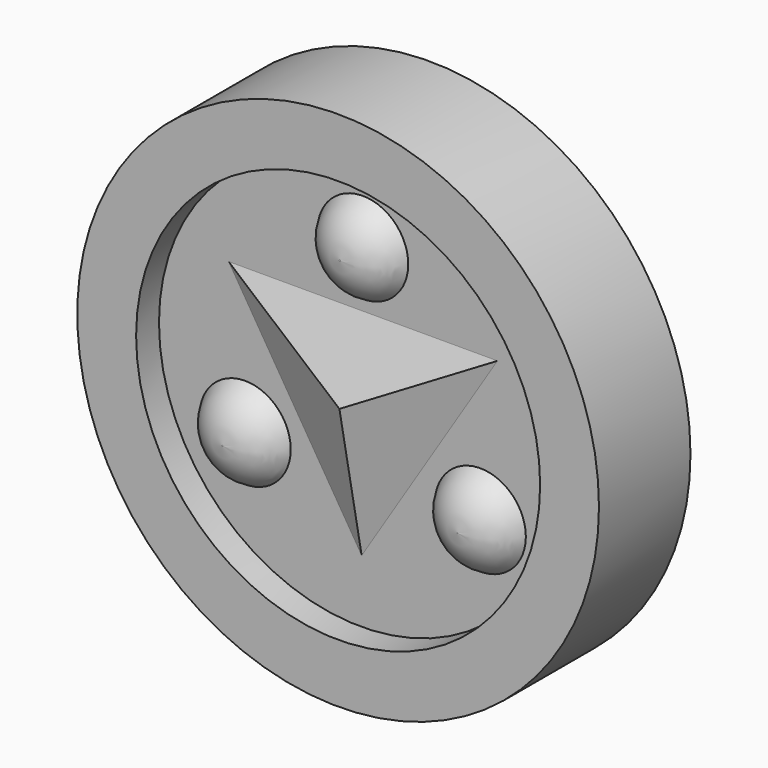
from build123d import *

# Parameters (mm, degrees)
F0_R          = 57.9269385224
F0_R_2        = 45.238930614
F0_R_3        = 10.232456426
F0_R_4        = 9.9260337363
F0_R_5        = 10.3400506536
F1_DEPTH      = 12.7
F2_DEPTH      = 12.7
F3_R          = 44.8601198224
F4_DEPTH      = 6.35
F5_R          = 44.7159015694
F6_DEPTH      = 6.35
F8_DEPTH      = 6.35
F10_DEPTH     = 6.35
F11_R         = 10.0879812564
F11_R_2       = 10.1077702508
F11_R_3       = 10.130036121
F12_DEPTH     = 6.35
F16_T4_DEPTH  = 143.3938123808
F16_T11_DEPTH = 146.5521785494
F16_T18_DEPTH = 143.0711301992


# Not quite as in the source:
# - a fillet or chamfer that OpenCascade refuses, or shapes differently, is made with other operations: its cross-section is extruded or revolved along the edge and cut away or added


with BuildPart() as f1:
    # F0 (on Front) → F1 (new body)
    with BuildSketch(Plane.XZ):
        Circle(F0_R)
        Circle(F0_R_2, mode=Mode.SUBTRACT)
        Circle(F0_R_2)
        with Locations((-26.1295642704, -15.3669575229)):
            Circle(F0_R_3, mode=Mode.SUBTRACT)
        Polygon((-12.544834055, -34.5090515912), (0, -5.3877583705), (12.6424450427, -34.5090515912), align=None, mode=Mode.SUBTRACT)
        with Locations((26.1333119124, -15.1850637048)):
            Circle(F0_R_4, mode=Mode.SUBTRACT)
        Polygon((-36.0336452723, 4.8764180392), (-24.01153557, 26.9035063684), (-4.5260344632, 1.7700339667), align=None, mode=Mode.SUBTRACT)
        Polygon((36.1581519246, 4.842239432), (4.4649434276, 1.758374623), (24.0084677935, 26.875147596), align=None, mode=Mode.SUBTRACT)
        with Locations((0, 29.5979101211)):
            Circle(F0_R_5, mode=Mode.SUBTRACT)
        with Locations((0, 29.5979101211)):
            Circle(F0_R_5)
        Polygon((-4.5260344632, 1.7700339667), (-24.01153557, 26.9035063684), (-36.0336452723, 4.8764180392), align=None)
        with Locations((-26.1295642704, -15.3669575229)):
            Circle(F0_R_3)
        Polygon((12.6424450427, -34.5090515912), (0, -5.3877583705), (-12.544834055, -34.5090515912), align=None)
        with Locations((26.1333119124, -15.1850637048)):
            Circle(F0_R_4)
        Polygon((24.0084677935, 26.875147596), (4.4649434276, 1.758374623), (36.1581519246, 4.842239432), align=None)
    extrude(amount=F1_DEPTH)

    # F2 (add): a face of the model
    f2_faces = [f1.faces().sort_by_distance(p)[0] for p in [
        (0, 0, 0),
    ]]
    extrude(f2_faces, amount=F2_DEPTH)

    # F3 (on face) → F4 (cut)
    with BuildSketch(Plane.XZ.offset(12.7)):
        Circle(F3_R)
    extrude(amount=-F4_DEPTH, mode=Mode.SUBTRACT)

    # F5 (on face) → F6 (cut)
    with BuildSketch(Plane(origin=(0, 12.7, 0), x_dir=(-1, 0, 0), z_dir=(0, 1, 0))):
        Circle(F5_R)
    extrude(amount=-F6_DEPTH, mode=Mode.SUBTRACT)

    # F7 (on face) → F8 (join)
    with BuildSketch(Plane(origin=(0, 6.35, 0), x_dir=(-1, 0, 0), z_dir=(0, 1, 0))):
        Polygon((0.1139463857, -15.4419038445), (-13.0555815995, 7.0367623121), (-26.1111631989, -15.4419038445), align=None)
        Polygon((0.1139463857, -15.4419038445), (13.1695279852, 7.0367623121), (-13.0555815995, 7.0367623121), align=None)
        Polygon((13.1695279852, 7.0367623121), (0, 29.5154284686), (-13.0555815995, 7.0367623121), align=None)
        Polygon((26.3390559703, -15.4419038445), (13.1695279852, 7.0367623121), (0.1139463857, -15.4419038445), align=None)
    extrude(amount=F8_DEPTH)

    # F9 (on face) → F10 (cut)
    with BuildSketch(Plane(origin=(0, 12.7, 0), x_dir=(-1, 0, 0), z_dir=(0, 1, 0))):
        Polygon((12.9840383306, 6.3451784663), (-12.7162076533, 6.3451784663), (0, -15.0037035346), align=None)
    extrude(amount=-F10_DEPTH, mode=Mode.SUBTRACT)

    # F11 (on face) → F12 (join)
    with BuildSketch(Plane.XZ.offset(6.35)):
        with Locations((0.4030804266, 29.4006802142)):
            Circle(F11_R)
        with Locations((26.4969747514, -15.3808789328)):
            Circle(F11_R_2)
        with Locations((-25.7336739451, -15.2944726869)):
            Circle(F11_R_3)
        Polygon((0.1468855771, -31.126530841), (30.5121447891, 17.0675422996), (-29.6086445451, 17.0675422996), align=None)
    extrude(amount=F12_DEPTH)

    # F13: fillet of radius 10.922 on 1 edges, made by hand

    # F13_s1 → F13_t2 (revolve, cut)
    with BuildSketch(Plane.XY.offset(29.4006802142)):
        with BuildLine():
            ThreePointArc((10.491061683, -6.35), (6.4607923392, -10.9765180328), (0.5720445946, -12.7))
            Line((0.5720445946, -12.7), (10.491061683, -12.7))
            Line((10.491061683, -12.7), (10.491061683, -6.35))
        make_face()
    revolve(axis=Axis((0.4030804266, -12.7, 29.4006802142), (0, -1, 0)), mode=Mode.SUBTRACT)

    # F14: fillet of radius 11.049 on 1 edges, made by hand

    # F14_s1 → F14_t2 (revolve, cut)
    with BuildSketch(Plane.XY.offset(-15.2944726869)):
        with BuildLine():
            ThreePointArc((-15.6036378241, -6.35), (-19.6807421254, -10.9783697257), (-25.6036278241, -12.7))
            Line((-25.6036278241, -12.7), (-15.6036378241, -12.7))
            Line((-15.6036378241, -12.7), (-15.6036378241, -6.35))
        make_face()
    revolve(axis=Axis((-25.7336739451, -12.7, -15.2944726869), (0, -1, 0)), mode=Mode.SUBTRACT)

    # F15: fillet of radius 11.049 on 1 edges, made by hand

    # F15_s1 → F15_t2 (revolve, cut)
    with BuildSketch(Plane.XY.offset(-15.3808789328)):
        with BuildLine():
            ThreePointArc((36.6047450022, -6.35), (32.5276407009, -10.9783697257), (26.6047550022, -12.7))
            Line((26.6047550022, -12.7), (36.6047450022, -12.7))
            Line((36.6047450022, -12.7), (36.6047450022, -6.35))
        make_face()
    revolve(axis=Axis((26.4969747514, -12.7, -15.3808789328), (0, -1, 0)), mode=Mode.SUBTRACT)

    # F16: chamfer of 16.6624 x 6.3960960974 on 3 edges, made by hand


with BuildPart() as f16_tool2:
    # F16_s3 → F16_t4 (new body)
    with BuildSketch(Plane(origin=(-37.0340982639, 0, -58.7784885341), x_dir=(0, 1, 0), z_dir=(0.5330752718, 0, 0.8460678191))):
        Polygon((-6.3039039026, -16.7170590485), (-12.7, -0.0546590485), (-12.7, -16.7170590485), align=None)
    extrude(amount=F16_T4_DEPTH)

    split(bisect_by=Plane.XZ.offset(6.35), keep=Keep.TOP)

    split(bisect_by=Plane.XY.offset(17.0675422996), keep=Keep.BOTTOM)

    split(bisect_by=Plane(origin=(-13.8075741275, 0, -8.5249421991), x_dir=(0, 1, 0), z_dir=(0.8508879508, 0, 0.5253472139)), keep=Keep.TOP)


with BuildPart() as f1_1:
    add(f1.part)

    # F16_t1: cut F16_tool2
    add(f16_tool2.part, mode=Mode.SUBTRACT)


with BuildPart() as f16_tool9:
    # F16_s10 → F16_t11 (new body)
    with BuildSketch(Plane.YZ.offset(73.7278393967)):
        Polygon((-6.3039039026, 17.0675422996), (-12.7, 0.4051422996), (-12.7, 17.0675422996), align=None)
    extrude(amount=-F16_T11_DEPTH)

    split(bisect_by=Plane.XZ.offset(6.35), keep=Keep.TOP)

    split(bisect_by=Plane(origin=(14.1437656916, 0, -8.9114507961), x_dir=(0, 1, 0), z_dir=(-0.8460678191, 0, 0.5330752718)), keep=Keep.TOP)

    split(bisect_by=Plane(origin=(-13.8075741275, 0, -8.5249421991), x_dir=(0, 1, 0), z_dir=(0.8508879508, 0, 0.5253472139)), keep=Keep.TOP)


with BuildPart() as f1_2:
    add(f1_1.part)

    # F16_t8: cut F16_tool9
    add(f16_tool9.part, mode=Mode.SUBTRACT)


with BuildPart() as f16_tool16:
    # F16_s17 → F16_t18 (new body)
    with BuildSketch(Plane(origin=(-38.5043151766, 0, 62.3641983265), x_dir=(0, 1, 0), z_dir=(0.5253472139, 0, -0.8508879508))):
        Polygon((-6.3039039026, -16.2272530881), (-12.7, 0.4351469119), (-12.7, -16.2272530881), align=None)
    extrude(amount=F16_T18_DEPTH)

    split(bisect_by=Plane.XZ.offset(6.35), keep=Keep.TOP)

    split(bisect_by=Plane(origin=(14.1437656916, 0, -8.9114507961), x_dir=(0, 1, 0), z_dir=(-0.8460678191, 0, 0.5330752718)), keep=Keep.TOP)

    split(bisect_by=Plane.XY.offset(17.0675422996), keep=Keep.BOTTOM)


with BuildPart() as f1_3:
    add(f1_2.part)

    # F16_t15: cut F16_tool16
    add(f16_tool16.part, mode=Mode.SUBTRACT)


solid = f1_3.part
